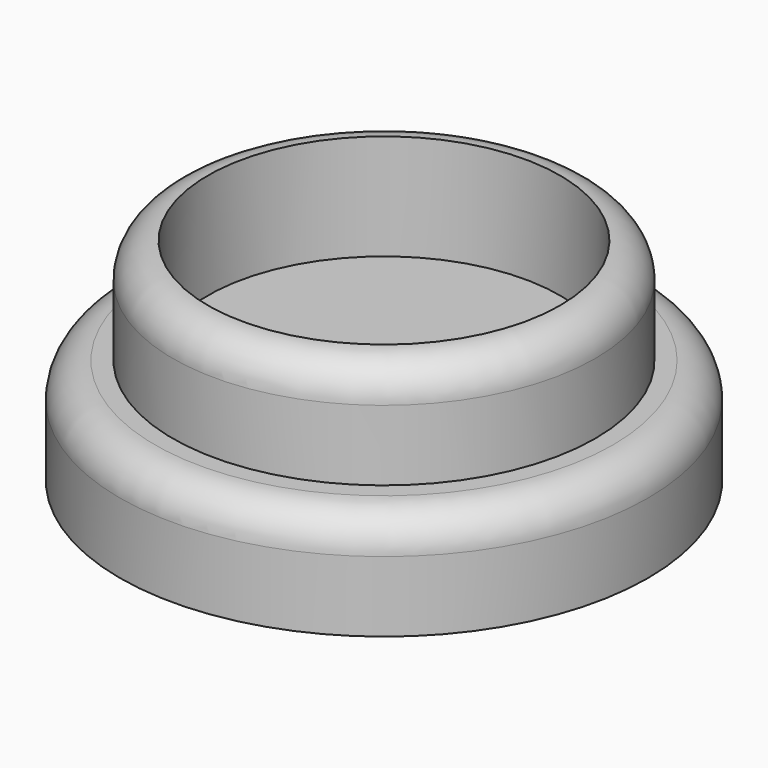
from build123d import *

# Parameters (mm, degrees)
F0_R     = 7.5
F0_R_2   = 6
F0_R_3   = 5
F1_DEPTH = 3
F2_DEPTH = 3
F3_R     = 0.99999


# Not quite as in the source:
# - a fillet or chamfer is up to 0.001 mm smaller than in the source, because OpenCascade refuses the exact size


with BuildPart() as f1:
    # F0 (on Top) → F1 (new body)
    with BuildSketch(Plane.XY):
        Circle(F0_R)
        Circle(F0_R_2, mode=Mode.SUBTRACT)
        Circle(F0_R_2)
        Circle(F0_R_3, mode=Mode.SUBTRACT)
        Circle(F0_R_3)
    extrude(amount=-F1_DEPTH)

    # F0 (on Top) → F2 (join)
    with BuildSketch(Plane.XY):
        Circle(F0_R_2)
        Circle(F0_R_3, mode=Mode.SUBTRACT)
    extrude(amount=F2_DEPTH)

    # F3 (radius 1 in the source; OpenCascade refuses exactly that, so slightly less here)
    f3_edges = [f1.edges().sort_by_distance(p)[0] for p in [
        (-7.5, 0, 0),
        (-6, 0, 3),
    ]]
    fillet(f3_edges, radius=F3_R)


solid = f1.part
